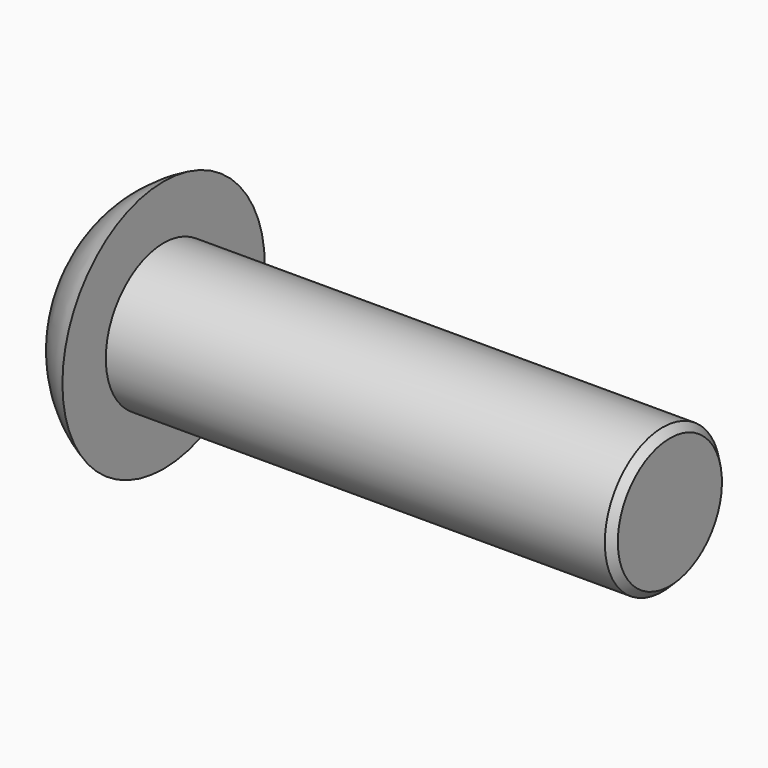
from build123d import *

# Parameters (mm, degrees)
F0_W     = 14
F0_H     = 2
F3_SIZE  = 0.2
F4_W     = 1.125
F4_H     = 1.5
F5_DEPTH = 15


# Not quite as in the source:
# - a fillet or chamfer that OpenCascade refuses, or shapes differently, is made with other operations: its cross-section is extruded or revolved along the edge and cut away or added


with BuildPart() as f1:
    # F0 (on Front) → F1 (revolve)
    with BuildSketch(Plane.XZ):
        with Locations((0.5, 1)):
            Rectangle(F0_W, F0_H)
        Polygon((-8.5, 0), (-6.5, 0), (-6.5, 2), (-6.5, 3.5), (-8.5, 3.5), align=None)
    revolve(axis=Axis((-0.5, 0, 0), (-1, 0, 0)))

    # F2: fillet of radius 3.5 on 1 edges, made by hand

    # F2_s1 → F2_t2 (revolve, cut)
    with BuildSketch(Plane.XZ):
        with BuildLine():
            ThreePointArc((-6.5, 3.5), (-7.9580398915, 2.2085510332), (-8.5, 0.3377223398))
            Line((-8.5, 0.3377223398), (-8.5, 3.5))
            Line((-8.5, 3.5), (-6.5, 3.5))
        make_face()
    revolve(axis=Axis((-8.5, 0, 0), (-1, 0, 0)), mode=Mode.SUBTRACT)

    # F3
    f3_edges = [f1.edges().sort_by_distance(p)[0] for p in [
        (7.5, 0, -2),
    ]]
    chamfer(f3_edges, length=F3_SIZE)

    # F4 (on face) → F5 (cut, symmetric)
    with BuildSketch(Plane.XZ):
        with Locations((-8.5627762601, 0)):
            Rectangle(F4_W, F4_H)
    extrude(amount=F5_DEPTH, both=True, mode=Mode.SUBTRACT)


solid = f1.part
